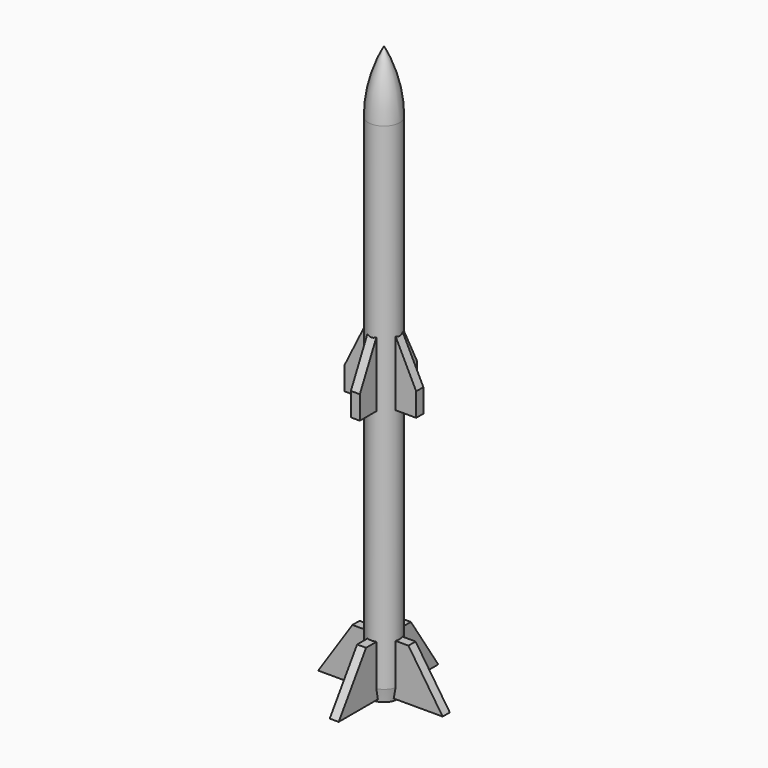
from build123d import *

# Parameters (mm, degrees)
F3_DEPTH = 0.2
F4_COUNT = 4


# Not quite as in the source:
# - a feature names something its author has since deleted; it is built from what else it names


with BuildPart() as f1:
    # F0 (on Front) → F1 (revolve)
    with BuildSketch(Plane.XZ):
        with BuildLine():
            Line((0, 25.4652777778), (0, 0))
            Line((0, 0), (0.6076388889, 0))
            Line((0.6076388889, 0), (0.7048611111, 0.5555555556))
            Line((0.7048611111, 0.5555555556), (0.7048611111, 22.6875))
            ThreePointArc((0.7048611111, 22.6875), (0.5258970546, 24.120406013), (0, 25.4652777778))
        make_face()
    revolve(axis=Axis((0, 0, 12.7326388889), (0, 0, 1)))

    # F2 (on Front) → F3 (join, symmetric)
    with BuildSketch(Plane.XZ):
        Polygon((0, 15.7317336792), (0, 11.4583333333), (1.5972222222, 11.4583333333), (1.5972222222, 12.5), align=None)
        Polygon((1.25, 2.3958333333), (0, 2.3958333333), (0, 0.5555555556), (0, 0.1041666667), (2.7777777778, 0.1041666667), align=None)
    extrude(amount=F3_DEPTH, both=True)

    # F4: F1 ×4 about axis
    f4_axis = Axis((0, 0, 0.5555555556), (0, 0, 1))


with BuildPart() as f1_1:
    add(f1.part)
    for i in range(1, F4_COUNT):
        add(f1.part.rotate(f4_axis, i * 360 / F4_COUNT))


solid = f1_1.part
